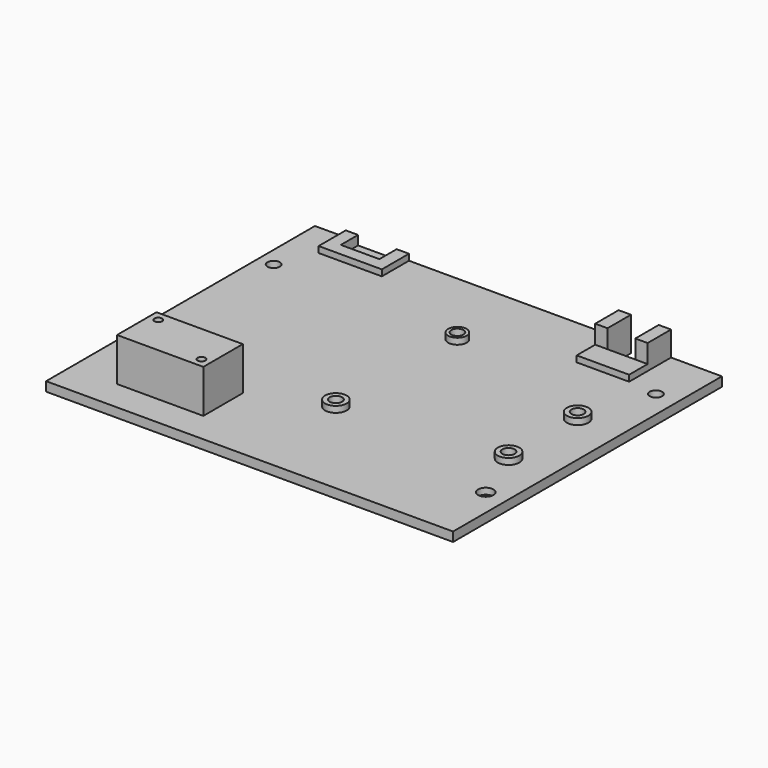
from build123d import *

# Parameters (mm, degrees)
F0_W      = 132
F0_H      = 109
F0_R      = 3.5
F0_R_2    = 2
F1_DEPTH  = 1
F2_W      = 132
F2_H      = 109
F2_R      = 3.5
F2_R_2    = 2
F2_R_3    = 2.5
F3_DEPTH  = 1
F4_R      = 2.5
F4_R_2    = 2
F5_DEPTH  = 1
F6_W      = 9
F6_H      = 9.5
F7_DEPTH  = 3
F8_R      = 3
F8_R_2    = 2
F8_R_3    = 3.5
F8_W      = 28
F8_H      = 16
F8_R_4    = 1.25
F9_DEPTH  = 2
F10_W     = 4
F10_H     = 9.5
F9_FACE_W = 28
F9_FACE_H = 16
F9_FACE_R = 1.25
F11_DEPTH = 6
F12_R     = 0.75
F13_DEPTH = 7
F14_W     = 28
F14_H     = 16
F14_R     = 1.25
F15_DEPTH = 6


# Not quite as in the source:
# - a feature names something its author has since deleted; it is built from what else it names


with BuildPart() as f1:
    # F0 (on Top) → F1 (new body)
    with BuildSketch(Plane.XY):
        with Locations((66, 54.5)):
            Rectangle(F0_W, F0_H)
        with Locations((5, 38)):
            Circle(F0_R, mode=Mode.SUBTRACT)
        with Locations((125, 22)):
            Circle(F0_R, mode=Mode.SUBTRACT)
        with Locations((66, 35)):
            Circle(F0_R_2, mode=Mode.SUBTRACT)
        with Locations((118, 40)):
            Circle(F0_R_2, mode=Mode.SUBTRACT)
        with Locations((5, 86)):
            Circle(F0_R_2, mode=Mode.SUBTRACT)
        with Locations((118, 68)):
            Circle(F0_R_2, mode=Mode.SUBTRACT)
        with Locations((67, 83)):
            Circle(F0_R_2, mode=Mode.SUBTRACT)
        with Locations((125, 91)):
            Circle(F0_R_2, mode=Mode.SUBTRACT)
    extrude(amount=F1_DEPTH)

    # F2 (on face) → F3 (join)
    with BuildSketch(Plane.XY.offset(1)):
        with Locations((66, 54.5)):
            Rectangle(F2_W, F2_H)
        with Locations((5, 38)):
            Circle(F2_R, mode=Mode.SUBTRACT)
        with Locations((125, 22)):
            Circle(F2_R, mode=Mode.SUBTRACT)
        with Locations((66, 35)):
            Circle(F2_R_2, mode=Mode.SUBTRACT)
        with Locations((118, 40)):
            Circle(F2_R_2, mode=Mode.SUBTRACT)
        with Locations((5, 86)):
            Circle(F2_R_2, mode=Mode.SUBTRACT)
        with Locations((118, 68)):
            Circle(F2_R_2, mode=Mode.SUBTRACT)
        with Locations((67, 83)):
            Circle(F2_R_2, mode=Mode.SUBTRACT)
        with Locations((125, 91)):
            Circle(F2_R_2, mode=Mode.SUBTRACT)
        with Locations((125, 22)):
            Circle(F2_R)
        with Locations((125, 22)):
            Circle(F2_R_3, mode=Mode.SUBTRACT)
        with Locations((5, 38)):
            Circle(F2_R)
        with Locations((5, 38)):
            Circle(F2_R_3, mode=Mode.SUBTRACT)
    extrude(amount=F3_DEPTH)

    # F4 (on face) → F5 (join)
    with BuildSketch(Plane.XY.offset(2)):
        Polygon((14, 102), (14, 109), (0, 109), (0, 0), (132, 0), (132, 109), (26.5, 109), (26.5, 102), align=None)
        with Locations((5, 38)):
            Circle(F4_R, mode=Mode.SUBTRACT)
        with Locations((125, 22)):
            Circle(F4_R, mode=Mode.SUBTRACT)
        with Locations((66, 35)):
            Circle(F4_R_2, mode=Mode.SUBTRACT)
        with Locations((118, 40)):
            Circle(F4_R_2, mode=Mode.SUBTRACT)
        with Locations((5, 86)):
            Circle(F4_R_2, mode=Mode.SUBTRACT)
        with Locations((118, 68)):
            Circle(F4_R_2, mode=Mode.SUBTRACT)
        with Locations((67, 83)):
            Circle(F4_R_2, mode=Mode.SUBTRACT)
        with Locations((125, 91)):
            Circle(F4_R_2, mode=Mode.SUBTRACT)
    extrude(amount=F5_DEPTH)

    # F6 (on face) → F7 (cut)
    with BuildSketch(Plane.XY.offset(3)):
        with Locations((107, 104.25)):
            Rectangle(F6_W, F6_H)
    extrude(amount=-F7_DEPTH, mode=Mode.SUBTRACT)

    # F8 (on face) → F9 (join)
    with BuildSketch(Plane.XY.offset(3)):
        Polygon((14, 102), (14, 109), (10, 109), (10, 98), (30.5, 98), (30.5, 109), (26.5, 109), (26.5, 102), align=None)
        Polygon((102.5, 109), (98.5, 109), (98.5, 92), (115.5, 92), (115.5, 109), (111.5, 109), (111.5, 99.5), (102.5, 99.5), align=None)
        with Locations((67, 83)):
            Circle(F8_R)
        with Locations((67, 83)):
            Circle(F8_R_2, mode=Mode.SUBTRACT)
        with Locations((66, 35)):
            Circle(F8_R_3)
        with Locations((66, 35)):
            Circle(F8_R_2, mode=Mode.SUBTRACT)
        with Locations((118, 68)):
            Circle(F8_R_3)
        with Locations((118, 68)):
            Circle(F8_R_2, mode=Mode.SUBTRACT)
        with Locations((118, 40)):
            Circle(F8_R_3)
        with Locations((118, 40)):
            Circle(F8_R_2, mode=Mode.SUBTRACT)
        with Locations((29, 18)):
            Rectangle(F8_W, F8_H)
        with Locations((18, 23)):
            Circle(F8_R_4, mode=Mode.SUBTRACT)
        with Locations((40, 13)):
            Circle(F8_R_4, mode=Mode.SUBTRACT)
    extrude(amount=F9_DEPTH)

    # F10 (on face) + F9_face (on face) → F11 (join)
    with BuildSketch(Plane.XY.offset(5)):
        with Locations((100.5, 104.25)):
            Rectangle(F10_W, F10_H)
        with Locations((113.5, 104.25)):
            Rectangle(F10_W, F10_H)
    with BuildSketch(Plane(origin=(67, 83, 5), x_dir=(1, 0, 0), z_dir=(0, 0, 1))):
        with Locations((-38, -65)):
            Rectangle(F9_FACE_W, F9_FACE_H)
        with Locations((-49, -60)):
            Circle(F9_FACE_R, mode=Mode.SUBTRACT)
        with Locations((-27, -70)):
            Circle(F9_FACE_R, mode=Mode.SUBTRACT)
    extrude(amount=F11_DEPTH)

    # F12 (on face) → F13 (cut)
    with BuildSketch(Plane(origin=(0, 99.5, 0), x_dir=(-1, 0, 0), z_dir=(0, 1, 0))):
        with Locations((-107, 3)):
            Circle(F12_R)
    extrude(amount=-F13_DEPTH, mode=Mode.SUBTRACT)

    # F14 (on face) → F15 (join)
    with BuildSketch(Plane.XY.offset(11)):
        with Locations((29, 18)):
            Rectangle(F14_W, F14_H)
        with Locations((40, 13)):
            Circle(F14_R, mode=Mode.SUBTRACT)
        with Locations((18, 23)):
            Circle(F14_R, mode=Mode.SUBTRACT)
    extrude(amount=F15_DEPTH)


solid = f1.part
